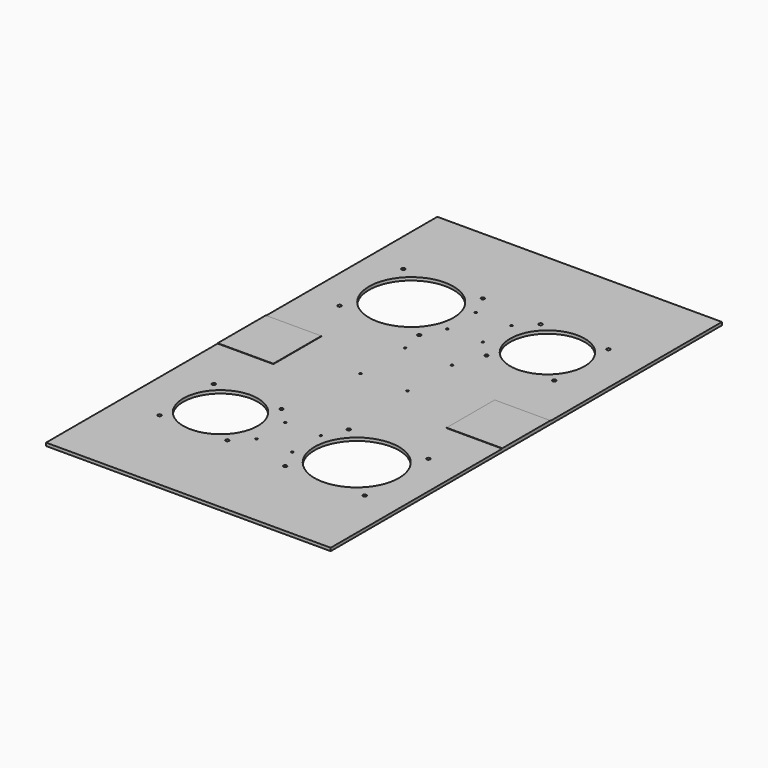
from build123d import *

# Parameters (mm, degrees)
F0_W     = 295.656
F0_H     = 508
F0_R     = 1.8288
F0_R_2   = 38.735
F0_R_3   = 43.8658
F1_DEPTH = 3.175
F2_W     = 57.8358
F2_H     = 62.3824
F3_DEPTH = 0.396875
F4_R     = 1.0922
F5_DEPTH = 3.175


# Not quite as in the source:
# - a length typed as a fraction of an inch, garbled in the dataset ("3 / 203.2 mm" for 3/8 in), is restored


with BuildPart() as f1:
    # F0 (on Top) → F1 (new body)
    with BuildSketch(Plane.XY):
        Rectangle(F0_W, F0_H)
        with Locations((-105.8926, -158.9786)):
            Circle(F0_R, mode=Mode.SUBTRACT)
        with Locations((-35.5854, -158.9786)):
            Circle(F0_R, mode=Mode.SUBTRACT)
        with Locations((-105.8926, -88.6714)):
            Circle(F0_R, mode=Mode.SUBTRACT)
        with Locations((-70.739, -123.825)):
            Circle(F0_R_2, mode=Mode.SUBTRACT)
        with Locations((-35.5854, -88.6714)):
            Circle(F0_R, mode=Mode.SUBTRACT)
        with Locations((29.39415, -165.16985)):
            Circle(F0_R, mode=Mode.SUBTRACT)
        with Locations((112.08385, -165.16985)):
            Circle(F0_R, mode=Mode.SUBTRACT)
        with Locations((29.39415, -82.48015)):
            Circle(F0_R, mode=Mode.SUBTRACT)
        with Locations((70.739, -123.825)):
            Circle(F0_R_3, mode=Mode.SUBTRACT)
        with Locations((112.08385, -82.48015)):
            Circle(F0_R, mode=Mode.SUBTRACT)
        with Locations((-112.08385, 82.48015)):
            Circle(F0_R, mode=Mode.SUBTRACT)
        with Locations((-70.739, 123.825)):
            Circle(F0_R_3, mode=Mode.SUBTRACT)
        with Locations((-29.39415, 82.48015)):
            Circle(F0_R, mode=Mode.SUBTRACT)
        with Locations((-112.08385, 165.16985)):
            Circle(F0_R, mode=Mode.SUBTRACT)
        with Locations((-29.39415, 165.16985)):
            Circle(F0_R, mode=Mode.SUBTRACT)
        with Locations((35.5854, 88.6714)):
            Circle(F0_R, mode=Mode.SUBTRACT)
        with Locations((70.739, 123.825)):
            Circle(F0_R_2, mode=Mode.SUBTRACT)
        with Locations((105.8926, 88.6714)):
            Circle(F0_R, mode=Mode.SUBTRACT)
        with Locations((35.5854, 158.9786)):
            Circle(F0_R, mode=Mode.SUBTRACT)
        with Locations((105.8926, 158.9786)):
            Circle(F0_R, mode=Mode.SUBTRACT)
    extrude(amount=F1_DEPTH)

    # F2 (on face) → F3 (join)
    with BuildSketch(Plane.XY.offset(3.175)):
        with Locations((118.9101, 0)):
            Rectangle(F2_W, F2_H)
        with Locations((-118.9101, 0)):
            Rectangle(F2_W, F2_H)
    extrude(amount=F3_DEPTH)

    # F4 (on face) → F5 (cut, through all)
    with BuildSketch(Plane.XY.offset(3.175)):
        with Locations((-24.3967, 0)):
            Circle(F4_R)
        with Locations((24.3967, 0)):
            Circle(F4_R)
        with Locations((-18.542, -105.283)):
            Circle(F4_R)
        with Locations((18.542, -105.283)):
            Circle(F4_R)
        with Locations((18.542, -142.367)):
            Circle(F4_R)
        with Locations((-18.542, -142.367)):
            Circle(F4_R)
        with Locations((-18.542, 142.367)):
            Circle(F4_R)
        with Locations((18.542, 142.367)):
            Circle(F4_R)
        with Locations((18.542, 105.283)):
            Circle(F4_R)
        with Locations((-18.542, 105.283)):
            Circle(F4_R)
        with Locations((-24.3967, 57.8612)):
            Circle(F4_R)
        with Locations((24.3967, 57.8612)):
            Circle(F4_R)
    extrude(amount=-F5_DEPTH, mode=Mode.SUBTRACT)


solid = f1.part
